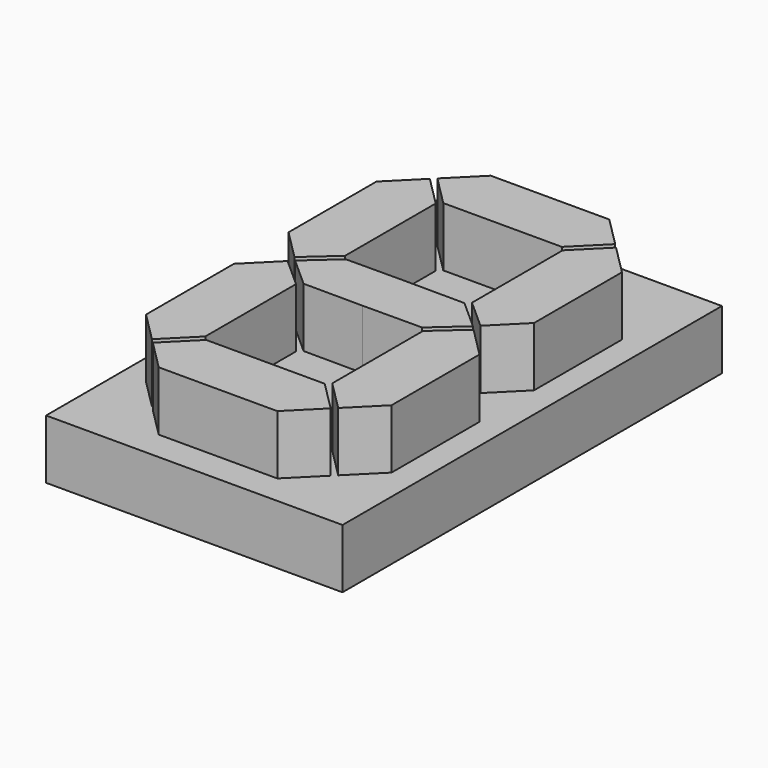
from build123d import *

# Parameters (mm, degrees)
F0_W     = 10
F0_H     = 16
F1_DEPTH = 2
F3_DEPTH = 2


# Not quite as in the source:
# - ends of sketch curves that miss each other by under 0.0002 mm in the source are joined


with BuildPart() as f1:
    # F0 (on Top) → F1 (new body)
    with BuildSketch(Plane.XY):
        Rectangle(F0_W, F0_H)
    extrude(amount=F1_DEPTH)

    # F2 (on face) → F3 (join)
    with BuildSketch(Plane.XY.offset(2)):
        Polygon((0, 7), (-2, 7), (-3, 6), (-2, 5), (0, 5), (2, 5), (3, 6), (2, 7), align=None)
        Polygon((-2.1414213562, 4.8585786438), (-3.1414213562, 5.8585786438), (-4.1414213562, 4.8585786438), (-4.1414213562, 1.1507223826), (-3.1374518146, 0.1453992321), (-2.1414213562, 1.0335195075), align=None)
        Polygon((2, 0.891659756), (2.00782e-05, 0.9006214721), (-2, 0.891659756), (-3, 0), (-2, -0.891659756), (-2.00782e-05, -0.9006214721), (2, -0.891659756), (3, 0), align=None)
        Polygon((0, -5), (-2, -5), (-3, -6), (-2, -7), (0, -7), (2, -7), (3, -6), (2, -5), align=None)
        Polygon((-4.1414213562, -4.8585786438), (-3.1414213562, -5.8585786438), (-2.1414213562, -4.8585786438), (-2.1414213562, -1.0335195075), (-3.1374518146, -0.1453992321), (-4.1414213562, -1.1507223826), align=None)
        Polygon((4.1414213562, 4.8585786438), (3.1414213562, 5.8585786438), (2.1414213562, 4.8585786438), (2.1414213562, 1.0335195075), (3.1374518146, 0.1453992321), (4.1414213562, 1.1507223826), align=None)
        Polygon((3.1374518146, -0.1453992321), (2.1414213562, -1.0335195075), (2.1414213562, -4.8585786438), (3.1414213562, -5.8585786438), (4.1414213562, -4.8585786438), (4.1414213562, -1.1507223826), align=None)
    extrude(amount=F3_DEPTH)


solid = f1.part
